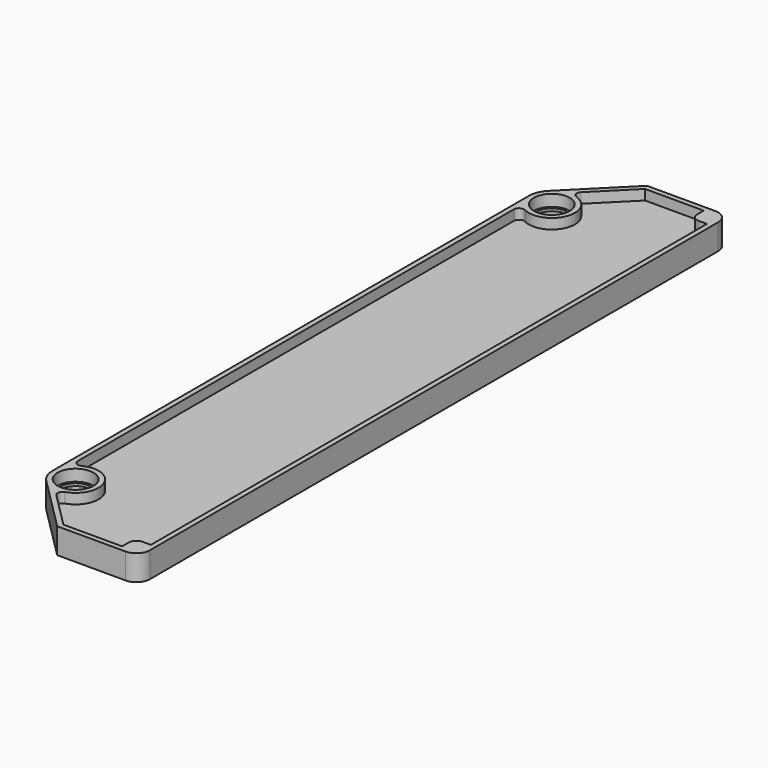
from build123d import *

# Parameters (mm, degrees)
F0_R      = 9.525
F1_DEPTH  = 15.8115
F2_R      = 11.1125
F3_DEPTH  = 7.112
F4_R      = 11.1125
F5_DEPTH  = 7.112
F6_T      = 3.175
F7_R      = 3.175
F8_DEPTH  = 3.175
F10_R     = 11.1125
F11_DEPTH = 1.5875
F12_W     = 13.096875
F12_H     = 13.096875
F13_DEPTH = 15.8115
F14_R     = 4.7625
F15_R     = 8.334375


# Not quite as in the source:
# - a shell that OpenCascade refuses in one call is made with other operations: the cavity is built on its own and cut out


with BuildPart() as f1:
    # F0 (on Top) → F1 (new body)
    with BuildSketch(Plane.XY):
        with BuildLine():
            Line((-14.2875, 369.1638474552), (-14.2875, 0))
            ThreePointArc((-14.2875, 0), (-13.1999288208, -5.4675895399), (-10.1027881362, -10.1027881362))
            Line((-10.1027881362, -10.1027881362), (23.8125, -44.0180762724))
            Line((23.8125, -44.0180762724), (74.6125, -44.0180762724))
            Line((74.6125, -44.0180762724), (74.6125, 413.1819237276))
            Line((74.6125, 413.1819237276), (23.8125, 413.1819237276))
            Line((23.8125, 413.1819237276), (-10.1027881362, 379.2666355914))
            ThreePointArc((-10.1027881362, 379.2666355914), (-13.1999288208, 374.6314369951), (-14.2875, 369.1638474552))
        make_face()
        Circle(F0_R, mode=Mode.SUBTRACT)
        with Locations((0, 369.1638474552)):
            Circle(F0_R, mode=Mode.SUBTRACT)
    extrude(amount=F1_DEPTH)

    # F2 (on face) → F3 (cut)
    with BuildSketch(Plane.XY.offset(15.8115)):
        with Locations((0, 369.1638474552)):
            Circle(F2_R)
        Circle(F2_R)
    extrude(amount=-F3_DEPTH, mode=Mode.SUBTRACT)

    # F4 (on face) → F5 (cut)
    with BuildSketch(Plane(origin=(0, 0, 0), x_dir=(1, 0, 0), z_dir=(0, 0, -1))):
        Circle(F4_R)
        with Locations((0, -369.1638474552)):
            Circle(F4_R)
    extrude(amount=-F5_DEPTH, mode=Mode.SUBTRACT)

    # F6: shell of thickness 3.175, made by hand


with BuildPart() as f6_core1:
    # F6_t2: copy of F1
    add(f1.part)

    # the walls: a layer under each face that stays
    f6_faces = [f6_core1.faces().sort_by_distance(p)[0] for p in [
        (-13.1999288208, 374.6314369951, 7.90575),
        (6.8548559319, 396.2242796595, 7.90575),
        (-14.2875, 184.5819237276, 7.90575),
        (30.1625, 184.5819237276, 15.8115),
        (49.2125, 413.1819237276, 7.90575),
        (-13.1999288208, -5.4675895399, 7.90575),
        (74.6125, 184.5819237276, 7.90575),
        (6.8548559319, -27.0604322043, 7.90575),
        (49.2125, -44.0180762724, 7.90575),
        (-11.1125, 0, 3.556),
        (-11.1125, 369.1638474552, 3.556),
        (-11.1125, 0, 12.2555),
        (-11.1125, 369.1638474552, 12.2555),
        (-7.4083333333, 7.4083333333, 7.112),
        (-7.4083333333, 376.5721807885, 7.112),
        (-7.4083333333, -7.4083333333, 8.6995),
        (-7.4083333333, 361.7555141219, 8.6995),
        (-9.525, 0, 7.90575),
        (-9.525, 369.1638474552, 7.90575),
    ]]
    thicken(f6_faces, amount=-F6_T, mode=Mode.SUBTRACT)

    # F6_s3 → F6_t4 (revolve, cut)
    with BuildSketch(Plane.XZ):
        Polygon((11.08075, 7.08025), (14.2875, 7.112), (14.2875, 10.287), (11.1125, 10.287), align=None)
    revolve(axis=Axis((0, 0, 7.112), (0, 0, -1)), mode=Mode.SUBTRACT)

    # F6_s5 → F6_t6 (revolve, cut)
    with BuildSketch(Plane.XZ.offset(-369.1638474552)):
        Polygon((11.08075, 7.08025), (14.2875, 7.112), (14.2875, 10.287), (11.1125, 10.287), align=None)
    revolve(axis=Axis((0, 369.1638474552, 7.112), (0, 0, -1)), mode=Mode.SUBTRACT)

    # F6_s7 → F6_t8 (revolve, cut)
    with BuildSketch(Plane.XZ):
        Polygon((11.08075, 8.73125), (14.2875, 8.6995), (14.2875, 5.5245), (11.1125, 5.5245), align=None)
    revolve(axis=Axis((0, 0, 8.6995), (0, 0, 1)), mode=Mode.SUBTRACT)

    # F6_s9 → F6_t10 (revolve, cut)
    with BuildSketch(Plane.XZ.offset(-369.1638474552)):
        Polygon((11.08075, 8.73125), (14.2875, 8.6995), (14.2875, 5.5245), (11.1125, 5.5245), align=None)
    revolve(axis=Axis((0, 369.1638474552, 8.6995), (0, 0, 1)), mode=Mode.SUBTRACT)


with BuildPart() as f1_1:
    add(f1.part)

    # what is left inside the walls is the cavity
    f6_cavity = [f6_core1.part.solids().sort_by_distance(p)[0] for p in [
        (30.1625, 109.440257, 12.60475),
    ]]
    add(f6_cavity, mode=Mode.SUBTRACT)

    # F7
    f7_edges = [f1_1.edges().sort_by_distance(p)[0] for p in [
        (-1.507724, 383.371572, 6.31825),
        (-11.1125, 360.183591, 6.31825),
        (-11.1125, 8.980256, 6.31825),
        (-1.507724, -14.207724, 6.31825),
    ]]
    fillet(f7_edges, radius=F7_R)

    # F8 (cut, through all): a face of the model
    f8_faces = [f1_1.faces().sort_by_distance(p)[0] for p in [
        (32.2546535053, 184.5819237276, 12.6365),
    ]]
    extrude(f8_faces, amount=-F8_DEPTH, mode=Mode.SUBTRACT)

    # F10 (on offset) → F11 (join, symmetric)
    with BuildSketch(Plane.XY.offset(7.90575)):
        with BuildLine():
            Line((74.6125, -44.0180762724), (74.6125, 413.1819237276))
            Line((74.6125, 413.1819237276), (23.8125, 413.1819237276))
            Line((23.8125, 413.1819237276), (-10.1027881362, 379.2666355914))
            ThreePointArc((-10.1027881362, 379.2666355914), (-13.1999288208, 374.6314369951), (-14.2875, 369.1638474552))
            Line((-14.2875, 369.1638474552), (-14.2875, 0))
            ThreePointArc((-14.2875, 0), (-13.1999288208, -5.4675895399), (-10.1027881362, -10.1027881362))
            Line((-10.1027881362, -10.1027881362), (23.8125, -44.0180762724))
            Line((23.8125, -44.0180762724), (74.6125, -44.0180762724))
        make_face()
        Circle(F10_R, mode=Mode.SUBTRACT)
        with Locations((0, 369.1638474552)):
            Circle(F10_R, mode=Mode.SUBTRACT)
    extrude(amount=F11_DEPTH, both=True)

    # F12 (on face) → F13 (join, through all)
    with BuildSketch(Plane(origin=(0, 0, 0), x_dir=(1, 0, 0), z_dir=(0, 0, -1))):
        with Locations((68.0640625, -406.6334862276)):
            Rectangle(F12_W, F12_H)
        with Locations((68.0640625, 37.4696387724)):
            Rectangle(F12_W, F12_H)
    extrude(amount=-F13_DEPTH)

    # F14
    f14_edges = [f1_1.edges().sort_by_distance(p)[0] for p in [
        (61.515625, 400.085049, 12.652375),
        (61.515625, 400.085049, 3.159125),
        (61.515625, -30.921201, 12.652375),
        (61.515625, -30.921201, 3.159125),
    ]]
    fillet(f14_edges, radius=F14_R)

    # F15
    f15_edges = [f1_1.edges().sort_by_distance(p)[0] for p in [
        (74.6125, -44.018076, 7.90575),
        (74.6125, 413.181924, 7.90575),
    ]]
    fillet(f15_edges, radius=F15_R)


solid = f1_1.part
